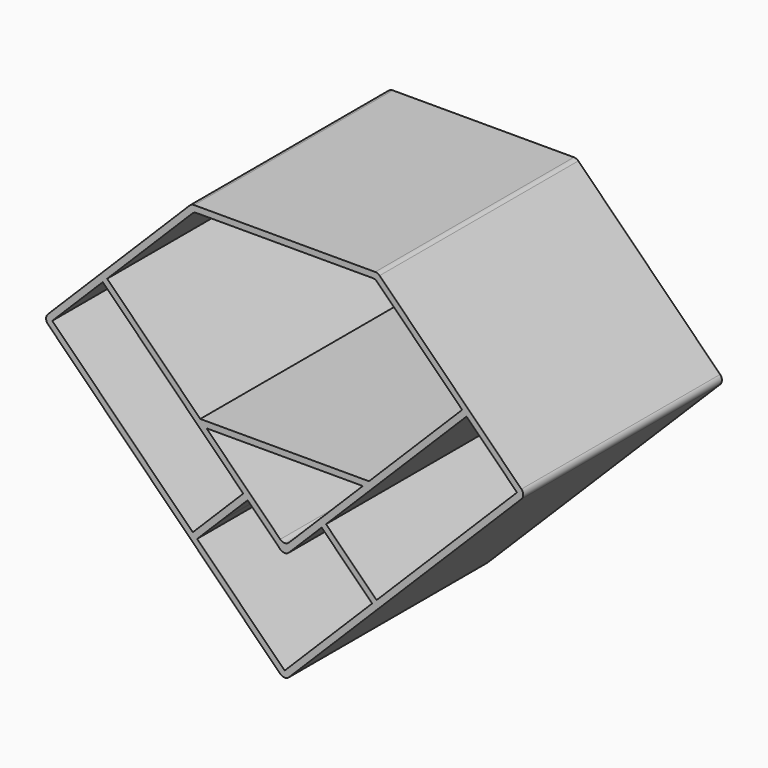
from build123d import *

# Parameters (mm, degrees)
F1_DEPTH = 400


# Not quite as in the source:
# - a feature names something its author has since deleted; it is built from what else it names


with BuildPart() as f1:
    # F0 (on Front) → F1 (new body)
    with BuildSketch(Plane.XZ):
        with BuildLine():
            Line((-292.9289321881, -7.0710678119), (-300, 0))
            Line((-300, 0), (-381.3172798365, -81.3172798365))
            ThreePointArc((-381.3172798365, -81.3172798365), (-384.2462120246, -88.3883476483), (-381.3172798365, -95.4594154602))
            Line((-381.3172798365, -95.4594154602), (-155.0431098568, -321.7335854399))
            ThreePointArc((-155.0431098568, -321.7335854399), (-147.9720420449, -324.662517628), (-140.900974233, -321.7335854399))
            Line((-140.900974233, -321.7335854399), (-103.7778682207, -284.6104794276))
            Line((-103.7778682207, -284.6104794276), (-59.5836943966, -240.4163056034))
            Line((-59.5836943966, -240.4163056034), (-66.6547622084, -233.3452377916))
            Line((-66.6547622085, -233.3452377916), (-147.9720420449, -314.662517628))
            Line((-147.9720420449, -314.662517628), (-374.2462120246, -88.3883476483))
            Line((-374.2462120246, -88.3883476483), (-292.9289321882, -7.0710678119))
        make_face()
        with BuildLine():
            Line((-152.9289321881, 147.0710678119), (-300, 0))
            Line((-300, 0), (-292.9289321881, -7.0710678119))
            Line((-292.9289321881, -7.0710678119), (-150, -150))
            Line((-150, -150), (-66.6547622084, -233.3452377916))
            Line((-66.6547622084, -233.3452377916), (-59.5836943966, -240.4163056034))
            Line((-59.5836943966, -240.4163056034), (-7.0710678119, -292.9289321881))
            ThreePointArc((-7.0710678119, -292.9289321881), (0, -295.8578643763), (7.0710678119, -292.9289321881))
            Line((7.0710678119, -292.9289321881), (59.5836943966, -240.4163056034))
            Line((59.5836943966, -240.4163056034), (66.6547622084, -233.3452377916))
            Line((66.6547622084, -233.3452377916), (150, -150))
            Line((150, -150), (225.0000048894, -74.9999951106))
            Line((225.0000048894, -74.9999951106), (292.9289321881, -7.0710678119))
            Line((292.9289321881, -7.0710678119), (300, 0))
            Line((300, 0), (152.9289321881, 147.0710678119))
            ThreePointArc((152.9289321881, 147.0710678119), (149.6846986999, 149.2387953251), (145.8578643763, 150))
            Line((145.8578643763, 150), (-145.8578643763, 150))
            ThreePointArc((-145.8578643763, 150), (-149.6846986999, 149.2387953251), (-152.9289321881, 147.0710678119))
        make_face()
        with BuildLine():
            ThreePointArc((7.0710678119, -278.7867965644), (0, -281.7157287525), (-7.0710678119, -278.7867965644))
            Line((-7.0710678119, -278.7867965644), (-125.8578643763, -160))
            Line((-125.8578643763, -160), (-135.8578643763, -150))
            Line((-135.8578643763, -150), (-210.8578643763, -75))
            Line((-210.8578643763, -75), (-285.8578643763, 0))
            Line((-285.8578643763, 0), (-148.7867965644, 137.0710678118))
            ThreePointArc((-148.7867965644, 137.0710678118), (-145.5425630762, 139.2387953251), (-141.7157287526, 140))
            Line((-141.7157287526, 140), (141.7157287525, 140))
            ThreePointArc((141.7157287525, 140), (145.5425630762, 139.2387953251), (148.7867965644, 137.0710678119))
            Line((148.7867965644, 137.0710678119), (285.8578643762, 0))
            Line((285.8578643762, 0), (210.8578643762, -75))
            Line((210.8578643762, -75), (135.8578643762, -150))
            Line((135.8578643762, -150), (125.8578643762, -160))
            Line((125.8578643762, -160), (7.0710678119, -278.7867965644))
        make_face(mode=Mode.SUBTRACT)
        with BuildLine():
            ThreePointArc((-140.900974233, -321.7335854399), (-147.9720420449, -324.662517628), (-155.0431098568, -321.7335854399))
            Line((-155.0431098568, -321.7335854399), (-7.0710678119, -469.7056274848))
            ThreePointArc((-7.0710678119, -469.7056274848), (0, -472.6345596729), (7.0710678119, -469.7056274848))
            Line((7.0710678119, -469.7056274848), (155.0431098568, -321.7335854399))
            ThreePointArc((155.0431098568, -321.7335854399), (147.9720420449, -324.662517628), (140.900974233, -321.7335854399))
            Line((140.900974233, -321.7335854399), (0, -462.6345596729))
            Line((0, -462.6345596729), (-140.900974233, -321.7335854399))
        make_face()
        with BuildLine():
            Line((381.3172798364, -81.3172798364), (300, 0))
            Line((300, 0), (292.9289321881, -7.0710678119))
            Line((292.9289321881, -7.0710678118), (374.2462120246, -88.3883476483))
            Line((374.2462120246, -88.3883476483), (147.9720420449, -314.662517628))
            Line((147.9720420449, -314.662517628), (66.6547622084, -233.3452377915))
            Line((66.6547622084, -233.3452377916), (59.5836943966, -240.4163056034))
            Line((59.5836943966, -240.4163056034), (140.900974233, -321.7335854399))
            ThreePointArc((140.900974233, -321.7335854399), (147.9720420449, -324.662517628), (155.0431098568, -321.7335854399))
            Line((155.0431098568, -321.7335854399), (381.3172798364, -95.4594154602))
            ThreePointArc((381.3172798364, -95.4594154602), (384.2462120246, -88.3883476483), (381.3172798364, -81.3172798364))
        make_face()
        Polygon((-135.8578643763, -150), (-125.8578643763, -160), (125.8578643762, -160), (135.8578643762, -150), align=None)
    extrude(amount=F1_DEPTH)


solid = f1.part
